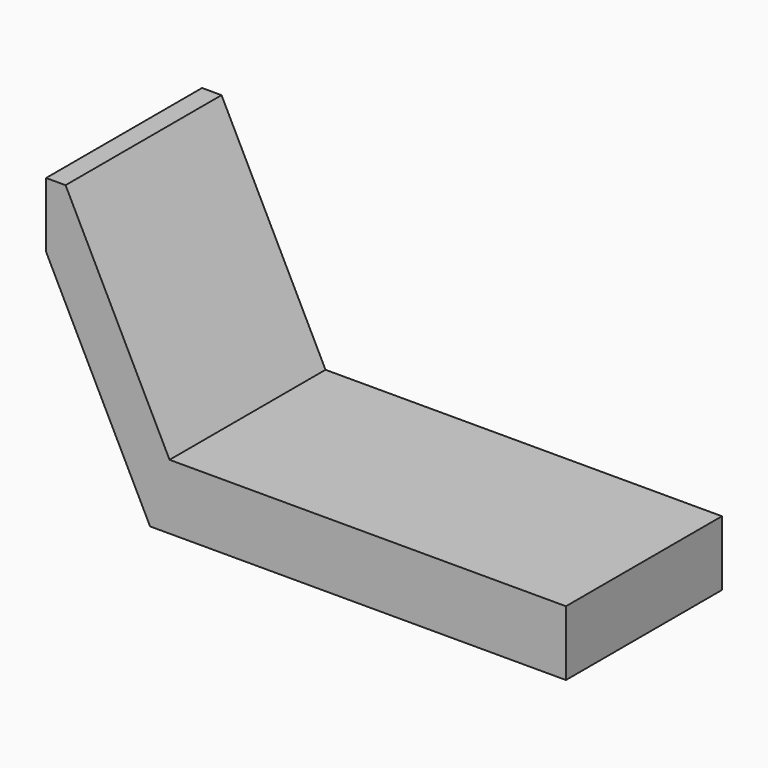
from build123d import *

# Parameters (mm, degrees)
F0_W     = 50.8
F0_H     = 6.35
F1_DEPTH = 19.05
F2_W     = 12.065
F2_H     = 19.05
F3_DEPTH = 20.32
F4_SIZE2 = 10.15999
F4_SIZE  = 20.31999
F5_SIZE2 = 20.32
F5_SIZE  = 10.16


# Not quite as in the source:
# - a fillet or chamfer is up to 0.001 mm smaller than in the source, because OpenCascade refuses the exact size


with BuildPart() as f1:
    # F0 (on Front) → F1 (new body)
    with BuildSketch(Plane.XZ):
        with Locations((-25.4, -3.175)):
            Rectangle(F0_W, F0_H)
    extrude(amount=F1_DEPTH)

    # F2 (on face) → F3 (join)
    with BuildSketch(Plane.XY):
        with Locations((-44.7675, -9.525)):
            Rectangle(F2_W, F2_H)
    extrude(amount=F3_DEPTH)

    # F4 (size 20.32 and 10.16 in the source; OpenCascade refuses exactly that, so slightly less here)
    f4_edges = [f1.edges().sort_by_distance(p)[0] for p in [
        (-38.735, -9.525, 20.32),
    ]]
    f4_side = f1.faces().sort_by_distance((-38.735, -9.525, 10.16))[0]
    chamfer(f4_edges, length=F4_SIZE, length2=F4_SIZE2, reference=f4_side)

    # F5
    f5_edges = [f1.edges().sort_by_distance(p)[0] for p in [
        (-50.8, -9.525, -6.35),
    ]]
    f5_side = f1.faces().sort_by_distance((-25.4, -9.525, -6.35))[0]
    chamfer(f5_edges, length=F5_SIZE, length2=F5_SIZE2, reference=f5_side)


solid = f1.part
